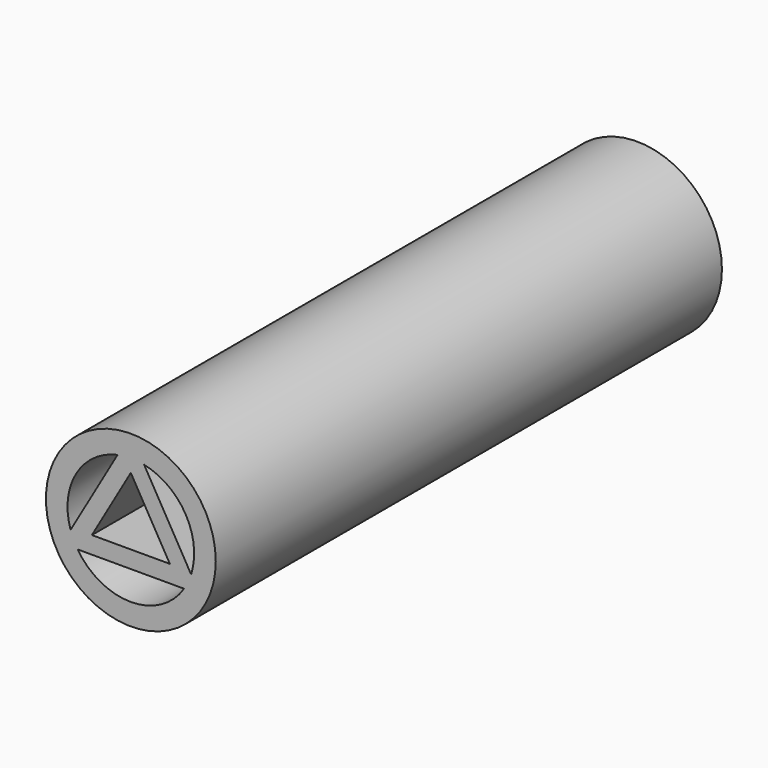
from build123d import *

# Parameters (mm, degrees)
F0_R     = 18.7507393172
F0_W     = 2.8121968498
F0_H     = 2.6235150942
F1_DEPTH = 139.7


# Not quite as in the source:
# - a feature names something its author has since deleted; it is built from what else it names


with BuildPart() as f1:
    # F0 (on Front) → F1 (new body)
    with BuildSketch(Plane.XZ):
        Circle(F0_R)
        with BuildLine():
            ThreePointArc((11.7463163557, -7.5817653145), (0, -13.9806692691), (-11.7463163557, -7.5817653145))
            Line((-11.7463163557, -7.5817653145), (11.7463163557, -7.5817653145))
        make_face(mode=Mode.SUBTRACT)
        with BuildLine():
            ThreePointArc((-13.3049026907, -4.2940281328), (-12.107614749, 6.9903346346), (-2.9337138978, 13.6693977914))
            Line((-2.9337138978, 13.6693977914), (-13.3049026907, -4.2940281328))
        make_face(mode=Mode.SUBTRACT)
        with Locations((-0.1412869315, 14.9811553385)):
            Rectangle(F0_W, F0_H, mode=Mode.SUBTRACT)
        Polygon((-8.6039650607, -3.7717653145), (0, 11.1307393172), (8.6039650607, -3.7717653145), align=None, mode=Mode.SUBTRACT)
        with BuildLine():
            ThreePointArc((2.9337138978, 13.6693977914), (12.107614749, 6.9903346346), (13.3049026907, -4.2940281328))
            Line((13.3049026907, -4.2940281328), (2.9337138978, 13.6693977914))
        make_face(mode=Mode.SUBTRACT)
        with Locations((-0.1412869315, 14.9811553385)):
            Rectangle(F0_W, F0_H)
    extrude(amount=F1_DEPTH)


solid = f1.part
